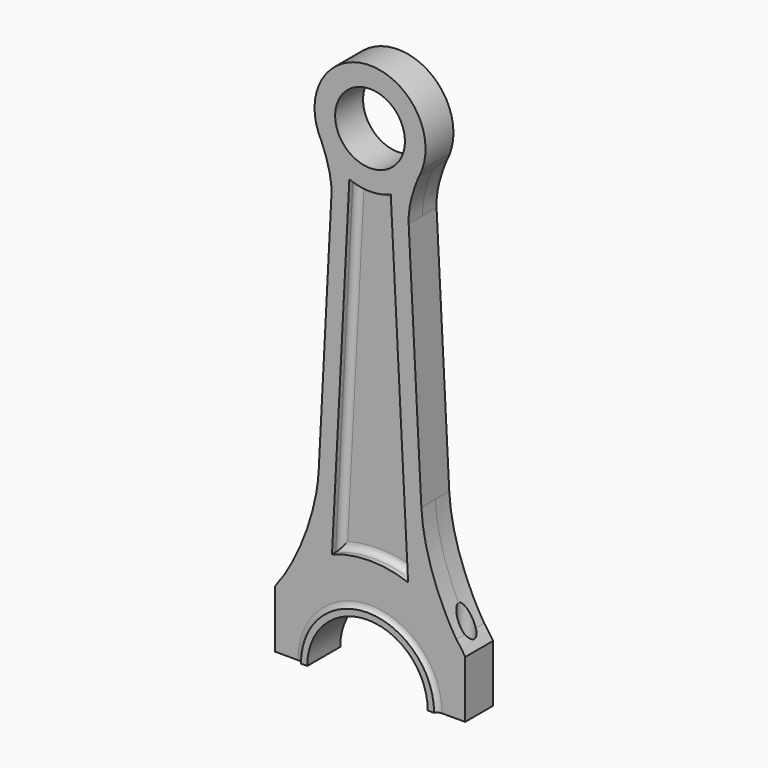
from build123d import *

# Parameters (mm, degrees)
F0_R         = 11
F1_DEPTH     = 5.5
F3_DEPTH     = 3.5
F5_DEPTH     = 3.5
F6_R         = 2.5
F7_DEPTH     = 42.164
F8_DEPTH     = 6.5
F9_T1_DEPTH  = 116.0281232172
F9_T3_DEPTH  = 116.0281232172
F9_T5_DEPTH  = 116.0281232172
F9_T7_DEPTH  = 116.0281232172
F9_T10_ANGLE = 180
F9_T12_ANGLE = 180
F9_T14_ANGLE = 56.4844529803
F9_T16_ANGLE = 76.5675906158
F9_T18_ANGLE = 76.5675906158
F9_T20_ANGLE = 56.4844529803


# Not quite as in the source:
# - a fillet or chamfer that OpenCascade refuses, or shapes differently, is made with other operations: its cross-section is extruded or revolved along the edge and cut away or added


with BuildPart() as f1:
    # F0 (on Front) → F1 (new body, symmetric)
    with BuildSketch(Plane.XZ):
        with BuildLine():
            ThreePointArc((-19, -33.2800959392), (0, -14.2800959392), (19, -33.2800959392))
            Line((19, -33.2800959392), (21, -33.2800959392))
            ThreePointArc((21, -33.2800959392), (0, -12.2800959392), (-21, -33.2800959392))
            Line((-21, -33.2800959392), (-19, -33.2800959392))
        make_face()
        with BuildLine():
            ThreePointArc((-21, -33.2800959392), (0, -12.2800959392), (21, -33.2800959392))
            Line((21, -33.2800959392), (30, -33.2800959392))
            Line((30, -33.2800959392), (30, -15.2523395618))
            add(Edge.make_bspline(
                [(27.2124389343, -11.2691176046), (28.1709489037, -12.7879287388), (29.112646753, -14.1276291325), (30, -15.2523395618)],
                knots=[33.1369304212, 33.1369304212, 33.1369304212, 33.1369304212, 39.5306887603, 39.5306887603, 39.5306887603, 39.5306887603], degree=3))
            ThreePointArc((27.2124389343, -11.2691176046), (22.7195127023, -6.6563519768), (17.4575728273, -2.9447510263))
            Line((17.4575728273, -2.9447510263), (16.1795605017, 21.7837348243))
            Line((16.1795605017, 21.7837348243), (12.1779068373, 99.2124372244))
            Line((12.1779068373, 99.2124372244), (11.6878243777, 108.6951291562))
            ThreePointArc((11.6878243777, 108.6951291562), (13.7183182045, 110.8544659363), (15.3552635835, 113.3255082945))
            add(Edge.make_bspline(
                [(15.3552635835, 113.3255082945), (15.770003684, 114.3065445088), (16.1590697648, 115.1520105897), (16.4735386522, 115.8146077708)],
                knots=[13.5101438027, 13.5101438027, 13.5101438027, 13.5101438027, 17.1488926622, 17.1488926622, 17.1488926622, 17.1488926622], degree=3))
            ThreePointArc((16.4735386522, 115.8146077708), (0, 139.2199040608), (-16.4735386522, 115.8146077708))
            add(Edge.make_bspline(
                [(-16.4735386522, 115.8146077708), (-16.1590697648, 115.1520105897), (-15.770003684, 114.3065445088), (-15.3552635835, 113.3255082945)],
                knots=[0, 0, 0, 0, 3.6387488595, 3.6387488595, 3.6387488595, 3.6387488595], degree=3))
            ThreePointArc((-15.3552635835, 113.3255082945), (-13.7183182045, 110.8544659363), (-11.6878243777, 108.6951291562))
            Line((-11.6878243777, 108.6951291562), (-12.1779068373, 99.2124372244))
            Line((-12.1779068373, 99.2124372244), (-16.1795605017, 21.7837348243))
            Line((-16.1795605017, 21.7837348243), (-17.4575728273, -2.9447510263))
            ThreePointArc((-17.4575728273, -2.9447510263), (-22.7195127023, -6.6563519768), (-27.2124389343, -11.2691176046))
            add(Edge.make_bspline(
                [(-30, -15.2523395618), (-29.112646753, -14.1276291325), (-28.1709489037, -12.7879287388), (-27.2124389343, -11.2691176046)],
                knots=[0, 0, 0, 0, 6.3937583391, 6.3937583391, 6.3937583391, 6.3937583391], degree=3))
            Line((-30, -15.2523395618), (-30, -33.2800959392))
            Line((-30, -33.2800959392), (-21, -33.2800959392))
        make_face()
        with Locations((0, 121.7199040608)):
            Circle(F0_R, mode=Mode.SUBTRACT)
        with BuildLine():
            add(Edge.make_bspline(
                [(27.2124389343, -11.2691176046), (28.1709489037, -12.7879287388), (29.112646753, -14.1276291325), (30, -15.2523395618)],
                knots=[33.1369304212, 33.1369304212, 33.1369304212, 33.1369304212, 39.5306887603, 39.5306887603, 39.5306887603, 39.5306887603], degree=3))
            ThreePointArc((30, -15.2523395618), (28.6754652359, -13.2122686152), (27.2124389343, -11.2691176046))
        make_face()
        with BuildLine():
            ThreePointArc((-27.2124389343, -11.2691176046), (-28.6754652359, -13.2122686152), (-30, -15.2523395618))
            add(Edge.make_bspline(
                [(-30, -15.2523395618), (-29.112646753, -14.1276291325), (-28.1709489037, -12.7879287388), (-27.2124389343, -11.2691176046)],
                knots=[0, 0, 0, 0, 6.3937583391, 6.3937583391, 6.3937583391, 6.3937583391], degree=3))
        make_face()
        with BuildLine():
            ThreePointArc((17.4575728273, -2.9447510263), (22.7195127023, -6.6563519768), (27.2124389343, -11.2691176046))
            add(Edge.make_bspline(
                [(16.1795605017, 21.7837348243), (16.8255200796, 9.2849490449), (22.2447694546, -3.3975753584), (27.2124389343, -11.2691176046)],
                knots=[0, 0, 0, 0, 33.1369304212, 33.1369304212, 33.1369304212, 33.1369304212], degree=3))
            Line((16.1795605017, 21.7837348243), (17.4575728273, -2.9447510263))
        make_face()
        with BuildLine():
            add(Edge.make_bspline(
                [(-27.2124389343, -11.2691176046), (-22.2447694546, -3.3975753584), (-16.8255200796, 9.2849490449), (-16.1795605017, 21.7837348243)],
                knots=[6.3937583391, 6.3937583391, 6.3937583391, 6.3937583391, 39.5306887603, 39.5306887603, 39.5306887603, 39.5306887603], degree=3))
            ThreePointArc((-27.2124389343, -11.2691176046), (-22.7195127023, -6.6563519768), (-17.4575728273, -2.9447510263))
            Line((-17.4575728273, -2.9447510263), (-16.1795605017, 21.7837348243))
        make_face()
        with BuildLine():
            Line((11.6878243777, 108.6951291562), (12.1779068373, 99.2124372244))
            add(Edge.make_bspline(
                [(12.1779068373, 99.2124372244), (11.9216008752, 104.1717464831), (13.8153940804, 109.6830639154), (15.3552635835, 113.3255082945)],
                knots=[0, 0, 0, 0, 13.5101438027, 13.5101438027, 13.5101438027, 13.5101438027], degree=3))
            ThreePointArc((15.3552635835, 113.3255082945), (13.7183182045, 110.8544659363), (11.6878243777, 108.6951291562))
        make_face()
        with BuildLine():
            add(Edge.make_bspline(
                [(-15.3552635835, 113.3255082945), (-13.8153940804, 109.6830639154), (-11.9216008752, 104.1717464831), (-12.1779068373, 99.2124372244)],
                knots=[3.6387488595, 3.6387488595, 3.6387488595, 3.6387488595, 17.1488926622, 17.1488926622, 17.1488926622, 17.1488926622], degree=3))
            Line((-12.1779068373, 99.2124372244), (-11.6878243777, 108.6951291562))
            ThreePointArc((-11.6878243777, 108.6951291562), (-13.7183182045, 110.8544659363), (-15.3552635835, 113.3255082945))
        make_face()
        with BuildLine():
            add(Edge.make_bspline(
                [(15.3552635835, 113.3255082945), (15.770003684, 114.3065445088), (16.1590697648, 115.1520105897), (16.4735386522, 115.8146077708)],
                knots=[13.5101438027, 13.5101438027, 13.5101438027, 13.5101438027, 17.1488926622, 17.1488926622, 17.1488926622, 17.1488926622], degree=3))
            ThreePointArc((15.3552635835, 113.3255082945), (15.9629905403, 114.5482283146), (16.4735386522, 115.8146077708))
        make_face()
        with BuildLine():
            ThreePointArc((-16.4735386522, 115.8146077708), (-15.9629905403, 114.5482283146), (-15.3552635835, 113.3255082945))
            add(Edge.make_bspline(
                [(-16.4735386522, 115.8146077708), (-16.1590697648, 115.1520105897), (-15.770003684, 114.3065445088), (-15.3552635835, 113.3255082945)],
                knots=[0, 0, 0, 0, 3.6387488595, 3.6387488595, 3.6387488595, 3.6387488595], degree=3))
        make_face()
    extrude(amount=F1_DEPTH, both=True)

    # F2 (on face) → F3 (cut)
    with BuildSketch(Plane.XZ.offset(5.5)):
        with BuildLine():
            ThreePointArc((6.5306906354, 105.4841386084), (0, 104.2199040608), (-6.5306906354, 105.4841386084))
            Line((-6.5306906354, 105.4841386084), (-12.0031098982, -0.4026667092))
            ThreePointArc((-12.0031098982, -0.4026667092), (0, 1.7199040608), (12.0031098982, -0.4026667092))
            Line((12.0031098982, -0.4026667092), (6.5306906354, 105.4841386084))
        make_face()
    extrude(amount=-F3_DEPTH, mode=Mode.SUBTRACT)

    # F4 (on face) → F5 (cut)
    with BuildSketch(Plane(origin=(0, 5.5, 0), x_dir=(-1, 0, 0), z_dir=(0, 1, 0))):
        with BuildLine():
            ThreePointArc((6.5306906354, 105.4841386084), (0, 104.2199040608), (-6.5306906354, 105.4841386084))
            Line((-6.5306906354, 105.4841386084), (-12.0031098982, -0.4026667092))
            ThreePointArc((-12.0031098982, -0.4026667092), (0, 1.7199040608), (12.0031098982, -0.4026667092))
            Line((12.0031098982, -0.4026667092), (6.5306906354, 105.4841386084))
        make_face()
    extrude(amount=-F5_DEPTH, mode=Mode.SUBTRACT)

    # F6 (on face) → F7 (cut)
    with BuildSketch(Plane(origin=(0, 0, -33.2800959392), x_dir=(1, 0, 0), z_dir=(0, 0, -1))):
        with Locations((-26, 0)):
            Circle(F6_R)
        with Locations((26, 0)):
            Circle(F6_R)
    extrude(amount=-F7_DEPTH, mode=Mode.SUBTRACT)

    # F0 (on Front) → F8 (join, symmetric)
    with BuildSketch(Plane.XZ):
        with BuildLine():
            ThreePointArc((-19, -33.2800959392), (0, -14.2800959392), (19, -33.2800959392))
            Line((19, -33.2800959392), (21, -33.2800959392))
            ThreePointArc((21, -33.2800959392), (0, -12.2800959392), (-21, -33.2800959392))
            Line((-21, -33.2800959392), (-19, -33.2800959392))
        make_face()
    extrude(amount=F8_DEPTH, both=True)

    # F9: fillet of radius 2 on 10 edges, made by hand

    # F9_s2 → F9_t1 (join)
    with BuildSketch(Plane(origin=(0.3107945998, 0, -6.0136195165), x_dir=(0, 1, 0), z_dir=(-0.0516129032, 0, 0.9986671659))):
        with BuildLine():
            ThreePointArc((-2, -9.966328946), (-2.5857864376, -11.3805425083), (-4, -11.966328946))
            Line((-4, -11.966328946), (-2, -11.966328946))
            Line((-2, -11.966328946), (-2, -9.966328946))
        make_face()
    extrude(amount=F9_T1_DEPTH)

    # F9_s4 → F9_t3 (join)
    with BuildSketch(Plane(origin=(5.6777536953, 0, 109.85985746), x_dir=(0, 1, 0), z_dir=(-0.0516129032, 0, -0.9986671659))):
        with BuildLine():
            ThreePointArc((-2, -9.966328946), (-2.5857864376, -11.3805425083), (-4, -11.966328946))
            Line((-4, -11.966328946), (-2, -11.966328946))
            Line((-2, -11.966328946), (-2, -9.966328946))
        make_face()
    extrude(amount=F9_T3_DEPTH)

    # F9_s6 → F9_t5 (join)
    with BuildSketch(Plane(origin=(-0.3107945998, 0, -6.0136195165), x_dir=(0, 1, 0), z_dir=(0.0516129032, 0, 0.9986671659))):
        with BuildLine():
            ThreePointArc((2, 9.966328946), (2.5857864376, 11.3805425083), (4, 11.966328946))
            Line((4, 11.966328946), (2, 11.966328946))
            Line((2, 11.966328946), (2, 9.966328946))
        make_face()
    extrude(amount=F9_T5_DEPTH)

    # F9_s8 → F9_t7 (join)
    with BuildSketch(Plane(origin=(-5.6777536953, 0, 109.85985746), x_dir=(0, 1, 0), z_dir=(0.0516129032, 0, -0.9986671659))):
        with BuildLine():
            ThreePointArc((4, 11.966328946), (2.5857864376, 11.3805425083), (2, 9.966328946))
            Line((2, 9.966328946), (2, 11.966328946))
            Line((2, 11.966328946), (4, 11.966328946))
        make_face()
    extrude(amount=F9_T7_DEPTH)

    # F9_s9 → F9_t10 (revolve)
    with BuildSketch(Plane.XY.offset(-33.2800959392)):
        with BuildLine():
            ThreePointArc((21, -6.5), (21.7320508076, -5.7679491924), (22.7320508076, -5.5))
            Line((22.7320508076, -5.5), (21, -5.5))
            Line((21, -5.5), (21, -6.5))
        make_face()
    revolve(axis=Axis((0, -5.5, -33.2800959392), (0, -1, 0)), revolution_arc=F9_T10_ANGLE)

    # F9_s11 → F9_t12 (revolve)
    with BuildSketch(Plane.XY.offset(-33.2800959392)):
        with BuildLine():
            ThreePointArc((22.7320508076, 5.5), (21.7320508076, 5.7679491924), (21, 6.5))
            Line((21, 6.5), (21, 5.5))
            Line((21, 5.5), (22.7320508076, 5.5))
        make_face()
    revolve(axis=Axis((0, 5.5, -33.2800959392), (0, -1, 0)), revolution_arc=F9_T12_ANGLE)

    # F9_s13 → F9_t14 (revolve)
    with BuildSketch(Plane(origin=(-13.8734074516, 0, -7.4520252165), x_dir=(0, 1, 0), z_dir=(-0.880954947, 0, -0.4732001494))):
        with BuildLine():
            ThreePointArc((-2, -7.6817348471), (-2.5857864376, -6.2675212848), (-4, -5.6817348471))
            Line((-4, -5.6817348471), (-2, -5.6817348471))
            Line((-2, -5.6817348471), (-2, -7.6817348471))
        make_face()
    revolve(axis=Axis((0, -2, -33.2800959392), (0, 1, 0)), revolution_arc=F9_T14_ANGLE)

    # F9_s15 → F9_t16 (revolve)
    with BuildSketch(Plane(origin=(59.1951057851, 0, 46.7222997417), x_dir=(0, 1, 0), z_dir=(0.7849516283, 0, 0.6195570525))):
        with BuildLine():
            ThreePointArc((-4, 78.044236888), (-2.5857864376, 77.4584504504), (-2, 76.044236888))
            Line((-2, 76.044236888), (-2, 78.044236888))
            Line((-2, 78.044236888), (-4, 78.044236888))
        make_face()
    revolve(axis=Axis((0, -2, 121.7199040608), (0, 1, 0)), revolution_arc=F9_T16_ANGLE)

    # F9_s17 → F9_t18 (revolve)
    with BuildSketch(Plane(origin=(-59.1951057851, 0, 46.7222997417), x_dir=(0, 1, 0), z_dir=(-0.7849516283, 0, 0.6195570525))):
        with BuildLine():
            ThreePointArc((2, -76.044236888), (2.5857864376, -77.4584504504), (4, -78.044236888))
            Line((4, -78.044236888), (2, -78.044236888))
            Line((2, -78.044236888), (2, -76.044236888))
        make_face()
    revolve(axis=Axis((0, 2, 121.7199040608), (0, -1, 0)), revolution_arc=F9_T18_ANGLE)

    # F9_s19 → F9_t20 (revolve)
    with BuildSketch(Plane(origin=(13.8734074516, 0, -7.4520252165), x_dir=(0, 1, 0), z_dir=(0.880954947, 0, -0.4732001494))):
        with BuildLine():
            ThreePointArc((2, 7.6817348471), (2.5857864376, 6.2675212848), (4, 5.6817348471))
            Line((4, 5.6817348471), (2, 5.6817348471))
            Line((2, 5.6817348471), (2, 7.6817348471))
        make_face()
    revolve(axis=Axis((0, 2, -33.2800959392), (0, -1, 0)), revolution_arc=F9_T20_ANGLE)


solid = f1.part
